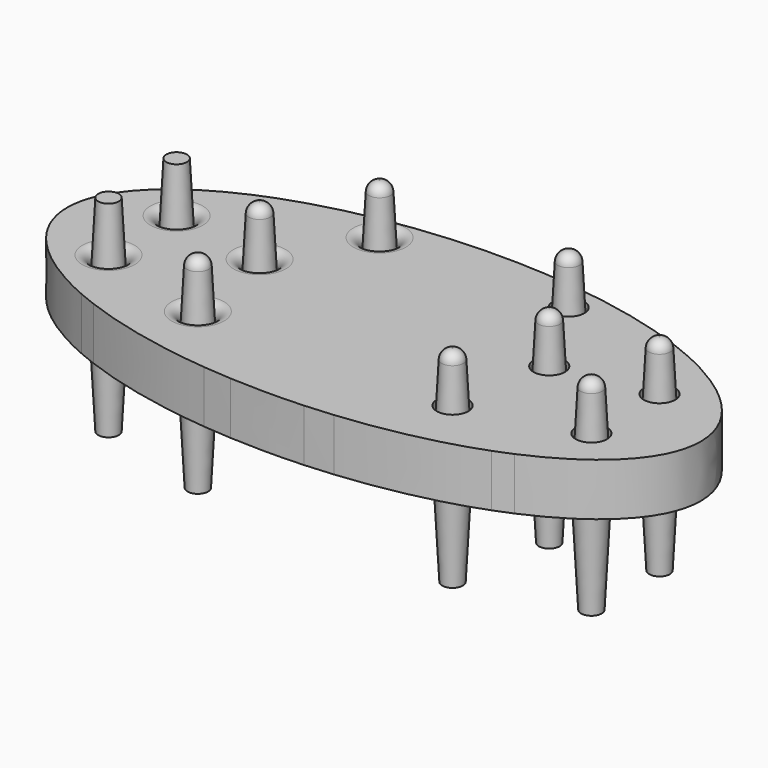
from build123d import *

# Parameters (mm, degrees)
F0_R     = 7.6143243375
F1_DEPTH = 25.4
F2_DEPTH = 49.8952651396
F2_TAPER = 3
F3_R     = 5.08
F3_2_R   = 5.08
F3_3_R   = 5.08
F3_4_R   = 5.08
F3_5_R   = 5.08
F3_6_R   = 5.08
F3_7_R   = 5.08
F3_8_R   = 5.08
F3_9_R   = 5.08


with BuildPart() as f1:
    # F0 (on Top) → F1 (new body)
    with BuildSketch(Plane.XY):
        with BuildLine():
            add(Edge.make_bspline(
                [(17.801263636, -70.8256252835), (24.6877059738, -70.4527018988), (31.4737791508, -69.7933493669)],
                knots=[4.8285294859, 4.8285294859, 4.8285294859, 4.9187327022, 4.9187327022, 4.9187327022], degree=2, weights=[1, 0.9989830949, 1]))
            ThreePointArc((31.4737791508, -69.7933493669), (31.8690856595, -68.424373517), (32.0024108255, -67.0057169295))
            ThreePointArc((32.0024108255, -67.0057169295), (22.41024302, -59.6527535587), (17.801263636, -70.8256252835))
        make_face()
        with BuildLine():
            add(Edge.make_bspline(
                [(-31.4737791508, -69.7933493669), (-24.6877059738, -70.4527018988), (-17.801263636, -70.8256252835)],
                knots=[4.5060452586, 4.5060452586, 4.5060452586, 4.5962484749, 4.5962484749, 4.5962484749], degree=2, weights=[1, 0.9989830949, 1]))
            ThreePointArc((-17.801263636, -70.8256252835), (-17.0351231172, -68.9835603975), (-16.7737621505, -67.0057169295))
            ThreePointArc((-16.7737621505, -67.0057169295), (-25.8067430755, -59.524717758), (-31.4737791508, -69.7933493669))
        make_face()
        with BuildLine():
            ThreePointArc((-7.6138200086, 71.2183590146), (0, 63.6916702477), (7.6138200086, 71.2183590146))
            add(Edge.make_bspline(
                [(7.6138200086, 71.2183590146), (0, 71.3937379931), (-7.6138200086, 71.2183590146)],
                knots=[1.5212128843, 1.5212128843, 1.5212128843, 1.6203797693, 1.6203797693, 1.6203797693], degree=2, weights=[1, 0.9987709929, 1]))
        make_face()
        with BuildLine():
            ThreePointArc((96.4467468907, 55.5009212788), (100.1127044041, 52.3824856248), (104.9164156319, 52.0854269475))
            add(Edge.make_bspline(
                [(104.9164156319, 52.0854269475), (100.816022601, 53.8650047926), (96.4467468907, 55.5009212788)],
                knots=[0.8189798537, 0.8189798537, 0.8189798537, 0.8920311964, 0.8920311964, 0.8920311964], degree=2, weights=[1, 0.9993330118, 1]))
        make_face()
        with BuildLine():
            ThreePointArc((-104.9164156319, 52.0854269475), (-100.1127044041, 52.3824856248), (-96.4467468907, 55.5009212788))
            add(Edge.make_bspline(
                [(-96.4467468907, 55.5009212788), (-100.816022601, 53.8650047926), (-104.9164156319, 52.0854269475)],
                knots=[2.2495614571, 2.2495614571, 2.2495614571, 2.3226127999, 2.3226127999, 2.3226127999], degree=2, weights=[1, 0.9993330118, 1]))
        make_face()
        with BuildLine():
            ThreePointArc((-96.4467468907, -55.5009212788), (-100.1127044041, -52.3824856248), (-104.9164156319, -52.0854269475))
            add(Edge.make_bspline(
                [(-104.9164156319, -52.0854269475), (-100.816022601, -53.8650047926), (-96.4467468907, -55.5009212788)],
                knots=[3.9605725073, 3.9605725073, 3.9605725073, 4.03362385, 4.03362385, 4.03362385], degree=2, weights=[1, 0.9993330118, 1]))
        make_face()
        with BuildLine():
            add(Edge.make_bspline(
                [(96.4467468907, -55.5009212788), (100.816022601, -53.8650047926), (104.9164156319, -52.0854269475)],
                knots=[5.3911541107, 5.3911541107, 5.3911541107, 5.4642054535, 5.4642054535, 5.4642054535], degree=2, weights=[1, 0.9993330118, 1]))
            ThreePointArc((104.9164156319, -52.0854269475), (100.1127044041, -52.3824856248), (96.4467468907, -55.5009212788))
        make_face()
        with BuildLine():
            add(Edge.make_bspline(
                [(104.9164156319, -52.0854269475), (153.6186337471, -30.9485779395), (153.6186337471, 0)],
                knots=[5.4642054535, 5.4642054535, 5.4642054535, 6.2831853072, 6.2831853072, 6.2831853072], degree=2, weights=[1, 0.9173240234, 1]))
            add(Edge.make_bspline(
                [(153.6186337471, 0), (153.6186337471, 30.9485779395), (104.9164156319, 52.0854269475)],
                knots=[0, 0, 0, 0.8189798537, 0.8189798537, 0.8189798537], degree=2, weights=[1, 0.9173240234, 1]))
            ThreePointArc((104.9164156319, 52.0854269475), (100.1127044041, 52.3824856248), (96.4467468907, 55.5009212788))
            add(Edge.make_bspline(
                [(96.4467468907, 55.5009212788), (57.5394135281, 70.0683581499), (7.6138200086, 71.2183590146)],
                knots=[0.8920311964, 0.8920311964, 0.8920311964, 1.5212128843, 1.5212128843, 1.5212128843], degree=2, weights=[1, 0.9509230626, 1]))
            ThreePointArc((7.6138200086, 71.2183590146), (0, 63.6916702477), (-7.6138200086, 71.2183590146))
            add(Edge.make_bspline(
                [(-7.6138200086, 71.2183590146), (-57.5394135281, 70.0683581499), (-96.4467468907, 55.5009212788)],
                knots=[1.6203797693, 1.6203797693, 1.6203797693, 2.2495614571, 2.2495614571, 2.2495614571], degree=2, weights=[1, 0.9509230626, 1]))
            ThreePointArc((-96.4467468907, 55.5009212788), (-100.1127044041, 52.3824856248), (-104.9164156319, 52.0854269475))
            add(Edge.make_bspline(
                [(-104.9164156319, 52.0854269475), (-224.9284298572, 0), (-104.9164156319, -52.0854269475)],
                knots=[2.3226127999, 2.3226127999, 2.3226127999, 3.9605725073, 3.9605725073, 3.9605725073], degree=2, weights=[1, 0.6829667279, 1]))
            ThreePointArc((-104.9164156319, -52.0854269475), (-100.1127044041, -52.3824856248), (-96.4467468907, -55.5009212788))
            add(Edge.make_bspline(
                [(-96.4467468907, -55.5009212788), (-67.6660249215, -66.2768165704), (-31.4737791508, -69.7933493669)],
                knots=[4.03362385, 4.03362385, 4.03362385, 4.5060452586, 4.5060452586, 4.5060452586], degree=2, weights=[1, 0.9722317246, 1]))
            ThreePointArc((-31.4737791508, -69.7933493669), (-25.8067430755, -59.524717758), (-16.7737621505, -67.0057169295))
            ThreePointArc((-16.7737621505, -67.0057169295), (-17.0351231172, -68.9835603975), (-17.801263636, -70.8256252835))
            add(Edge.make_bspline(
                [(-17.801263636, -70.8256252835), (0, -71.7896219543), (17.801263636, -70.8256252835)],
                knots=[4.5962484749, 4.5962484749, 4.5962484749, 4.8285294859, 4.8285294859, 4.8285294859], degree=2, weights=[1, 0.993263269, 1]))
            ThreePointArc((17.801263636, -70.8256252835), (22.41024302, -59.6527535587), (32.0024108255, -67.0057169295))
            ThreePointArc((32.0024108255, -67.0057169295), (31.8690856595, -68.424373517), (31.4737791508, -69.7933493669))
            add(Edge.make_bspline(
                [(31.4737791508, -69.7933493669), (67.6660249215, -66.2768165704), (96.4467468907, -55.5009212788)],
                knots=[4.9187327022, 4.9187327022, 4.9187327022, 5.3911541107, 5.3911541107, 5.3911541107], degree=2, weights=[1, 0.9722317246, 1]))
            ThreePointArc((96.4467468907, -55.5009212788), (100.1127044041, -52.3824856248), (104.9164156319, -52.0854269475))
        make_face()
        with Locations((-117.0822919246, -20.6447670295)):
            Circle(F0_R, mode=Mode.SUBTRACT)
        with Locations((-61.7528027529, -35.6529972926)):
            Circle(F0_R, mode=Mode.SUBTRACT)
        with Locations((61.7528027529, -35.6529972926)):
            Circle(F0_R, mode=Mode.SUBTRACT)
        with Locations((117.0822919246, -20.6447670295)):
            Circle(F0_R, mode=Mode.SUBTRACT)
        with Locations((-117.0822919246, 20.6447670295)):
            Circle(F0_R, mode=Mode.SUBTRACT)
        with Locations((-70.2226963037, 12.3821560164)):
            Circle(F0_R, mode=Mode.SUBTRACT)
        with Locations((-45.8346098157, 54.6235609131)):
            Circle(F0_R, mode=Mode.SUBTRACT)
        with Locations((70.2226963037, 12.3821560164)):
            Circle(F0_R, mode=Mode.SUBTRACT)
        with Locations((45.8346098157, 54.6235609131)):
            Circle(F0_R, mode=Mode.SUBTRACT)
        with Locations((117.0822919246, 20.6447670295)):
            Circle(F0_R, mode=Mode.SUBTRACT)
    extrude(amount=F1_DEPTH)

    # F3
    f3_edges = [f1.edges().sort_by_distance(p)[0] for p in [
        (-124.696616, 20.644767, 25.4),
        (-124.696616, -20.644767, 25.4),
        (-69.367127, -35.652997, 25.4),
        (-77.837021, 12.382156, 25.4),
        (-53.448934, 54.623561, 25.4),
    ]]
    fillet(f3_edges, radius=F3_R)


with BuildPart() as f2:
    # F0 (on Top) → F2 (new body, symmetric)
    with BuildSketch(Plane.XY):
        with Locations((-117.0822919246, 20.6447670295)):
            Circle(F0_R)
    extrude(amount=F2_DEPTH, both=True, taper=F2_TAPER)


with BuildPart() as f2b:
    # F0 (on Top) → F2, piece 2 (new body, symmetric)
    with BuildSketch(Plane.XY):
        with Locations((-117.0822919246, -20.6447670295)):
            Circle(F0_R)
    extrude(amount=F2_DEPTH, both=True, taper=F2_TAPER)


with BuildPart() as f2c:
    # F0 (on Top) → F2, piece 3 (new body, symmetric)
    with BuildSketch(Plane.XY):
        with Locations((-61.7528027529, -35.6529972926)):
            Circle(F0_R)
    extrude(amount=F2_DEPTH, both=True, taper=F2_TAPER)

    # F3#2
    f3_2_edges = [f2c.edges().sort_by_distance(p)[0] for p in [
        (-66.752227, -35.652997, 49.895265),
    ]]
    fillet(f3_2_edges, radius=F3_2_R)


with BuildPart() as f2d:
    # F0 (on Top) → F2, piece 4 (new body, symmetric)
    with BuildSketch(Plane.XY):
        with Locations((-70.2226963037, 12.3821560164)):
            Circle(F0_R)
    extrude(amount=F2_DEPTH, both=True, taper=F2_TAPER)

    # F3#3
    f3_3_edges = [f2d.edges().sort_by_distance(p)[0] for p in [
        (-75.222121, 12.382156, 49.895265),
    ]]
    fillet(f3_3_edges, radius=F3_3_R)


with BuildPart() as f2e:
    # F0 (on Top) → F2, piece 5 (new body, symmetric)
    with BuildSketch(Plane.XY):
        with Locations((-45.8346098157, 54.6235609131)):
            Circle(F0_R)
    extrude(amount=F2_DEPTH, both=True, taper=F2_TAPER)

    # F3#4
    f3_4_edges = [f2e.edges().sort_by_distance(p)[0] for p in [
        (-50.834034, 54.623561, 49.895265),
    ]]
    fillet(f3_4_edges, radius=F3_4_R)


with BuildPart() as f2f:
    # F0 (on Top) → F2, piece 6 (new body, symmetric)
    with BuildSketch(Plane.XY):
        with Locations((45.8346098157, 54.6235609131)):
            Circle(F0_R)
    extrude(amount=F2_DEPTH, both=True, taper=F2_TAPER)

    # F3#5
    f3_5_edges = [f2f.edges().sort_by_distance(p)[0] for p in [
        (40.835186, 54.623561, 49.895265),
    ]]
    fillet(f3_5_edges, radius=F3_5_R)


with BuildPart() as f2g:
    # F0 (on Top) → F2, piece 7 (new body, symmetric)
    with BuildSketch(Plane.XY):
        with Locations((70.2226963037, 12.3821560164)):
            Circle(F0_R)
    extrude(amount=F2_DEPTH, both=True, taper=F2_TAPER)

    # F3#6
    f3_6_edges = [f2g.edges().sort_by_distance(p)[0] for p in [
        (65.223272, 12.382156, 49.895265),
    ]]
    fillet(f3_6_edges, radius=F3_6_R)


with BuildPart() as f2h:
    # F0 (on Top) → F2, piece 8 (new body, symmetric)
    with BuildSketch(Plane.XY):
        with Locations((61.7528027529, -35.6529972926)):
            Circle(F0_R)
    extrude(amount=F2_DEPTH, both=True, taper=F2_TAPER)

    # F3#7
    f3_7_edges = [f2h.edges().sort_by_distance(p)[0] for p in [
        (56.753378, -35.652997, 49.895265),
    ]]
    fillet(f3_7_edges, radius=F3_7_R)


with BuildPart() as f2i:
    # F0 (on Top) → F2, piece 9 (new body, symmetric)
    with BuildSketch(Plane.XY):
        with Locations((117.0822919246, -20.6447670295)):
            Circle(F0_R)
    extrude(amount=F2_DEPTH, both=True, taper=F2_TAPER)

    # F3#8
    f3_8_edges = [f2i.edges().sort_by_distance(p)[0] for p in [
        (112.082868, -20.644767, 49.895265),
    ]]
    fillet(f3_8_edges, radius=F3_8_R)


with BuildPart() as f2j:
    # F0 (on Top) → F2, piece 10 (new body, symmetric)
    with BuildSketch(Plane.XY):
        with Locations((117.0822919246, 20.6447670295)):
            Circle(F0_R)
    extrude(amount=F2_DEPTH, both=True, taper=F2_TAPER)

    # F3#9
    f3_9_edges = [f2j.edges().sort_by_distance(p)[0] for p in [
        (112.082868, 20.644767, 49.895265),
    ]]
    fillet(f3_9_edges, radius=F3_9_R)


solid = Compound([f1.part, f2.part, f2b.part, f2c.part, f2d.part, f2e.part, f2f.part, f2g.part, f2h.part, f2i.part, f2j.part])
